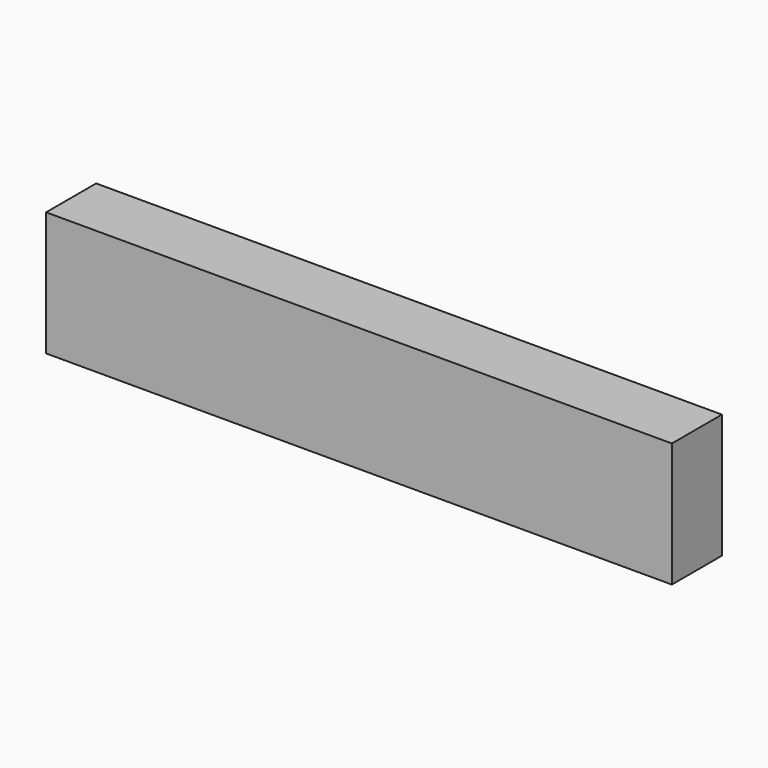
from build123d import *

# Parameters (mm, degrees)
F1_E1_RIGHT_W = 50.4280775785
F1_E1_RIGHT_H = 25.4
F2_DEPTH      = 254


with BuildPart() as f2:
    # F1_E1_right (on explicit) → F2 (new body)
    with BuildSketch(Plane(origin=(27.0196869969, 0, 0), x_dir=(0, 0, 1), z_dir=(1, 0, 0))):
        with Locations((25.2140387893, 12.7)):
            Rectangle(F1_E1_RIGHT_W, F1_E1_RIGHT_H)
    extrude(amount=F2_DEPTH)


solid = f2.part
